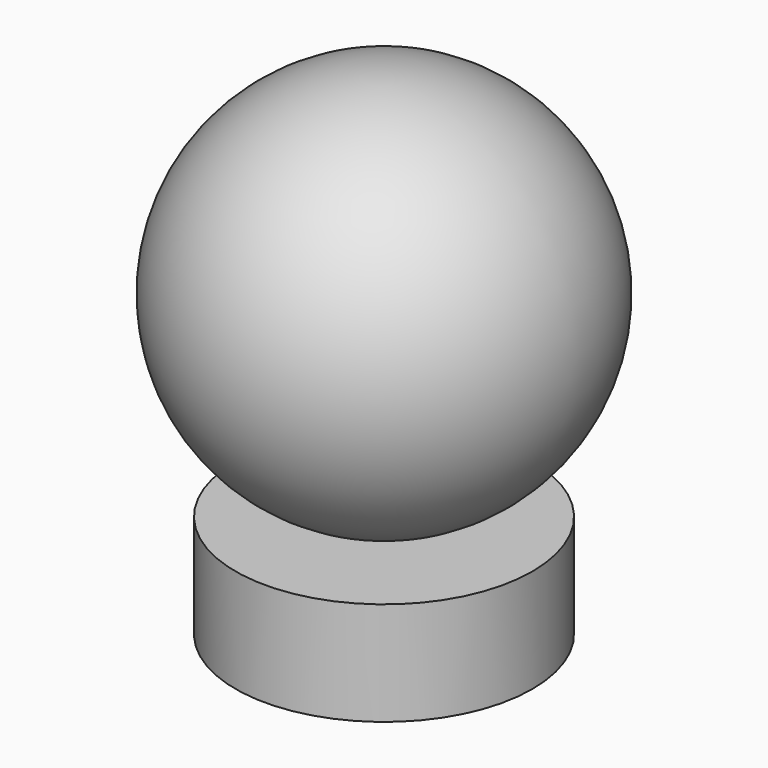
from build123d import *

# Parameters (mm, degrees)
F3_R     = 9.75
F4_DEPTH = 6.8


# Not quite as in the source:
# - the program builds the solid bodies; features that only make, move or delete a surface that nothing else refers to are left out


with BuildPart() as f1:
    # F0 (on Front) → F1 (revolve)
    with BuildSketch(Plane.XZ):
        with BuildLine():
            Line((0, 32.4), (0, 7))
            ThreePointArc((0, 7), (12.7, 19.7), (0, 32.4))
        make_face()
    revolve(axis=Axis((0, 0, 19.7), (0, 0, -1)))


with BuildPart() as f4:
    # F3 (on Top) → F4 (new body)
    with BuildSketch(Plane.XY):
        Circle(F3_R)
    extrude(amount=F4_DEPTH)


solid = Compound([f1.part, f4.part])
